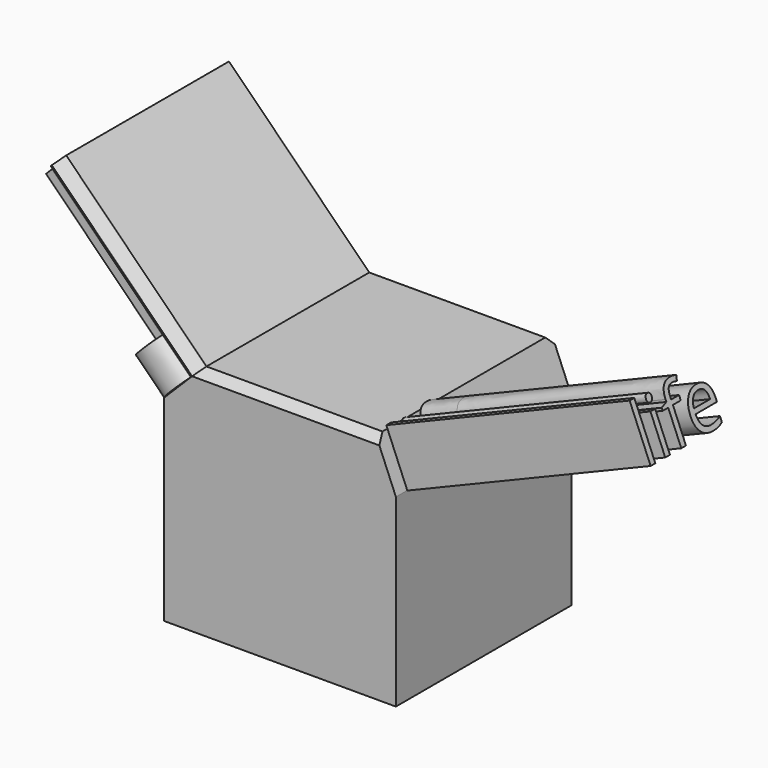
from build123d import *

# Parameters (mm, degrees)
F0_W         = 147.5178673863
F0_H         = 148.0135470629
F1_DEPTH     = 139.7
F2_SIZE      = 22.86
F3_SIZE      = 5.08
F4_TEXT_SIZE = 44.9012806053
F5_DEPTH     = 25.4
F6_T1_DEPTH  = 271.4076559597
F7_TEXT_SIZE = 46.0137451665
F8_DEPTH     = 25.4
F9_DEPTH     = 167.64
F10_DEPTH    = 126.238


# Not quite as in the source:
# - a fillet or chamfer that OpenCascade refuses, or shapes differently, is made with other operations: its cross-section is extruded or revolved along the edge and cut away or added
# - Text() gives the source's letters only with a copy of the font that has no kerning and outlines rounded to 1/6400 em; it was checked with that copy


with BuildPart() as f1:
    # F0 (on Front) → F1 (new body)
    with BuildSketch(Plane.XZ):
        with Locations((-1.3054646552, 0.765427947)):
            Rectangle(F0_W, F0_H)
    extrude(amount=F1_DEPTH)

    # F2
    f2_edges = [f1.edges().sort_by_distance(p)[0] for p in [
        (-75.064398, -69.85, 74.772201),
    ]]
    chamfer(f2_edges, length=F2_SIZE)

    # F3
    f3_edges = [f1.edges().sort_by_distance(p)[0] for p in [
        (10.124535, 0, 74.772201),
        (72.453469, -69.85, 74.772201),
        (10.124535, -139.7, 74.772201),
    ]]
    chamfer(f3_edges, length=F3_SIZE)

    # F4 (on face) → F5 (join)
    with BuildSketch(Plane(origin=(-63.4882999134, 0, 63.4882999134), x_dir=(0, -1, 0), z_dir=(-0.7071067812, 0, 0.7071067812))):
        with Locations((5.08, -16.371075406)):
            Text('trump', F4_TEXT_SIZE, font='Open Sans', font_style=FontStyle.BOLD, text_align=(TextAlign.LEFT, TextAlign.BOTTOM))
    extrude(amount=F5_DEPTH)

    # F6: chamfer of 25.4 on 1 edges, made by hand

    # F6_s2 → F6_t1 (cut)
    with BuildSketch(Plane.XZ.offset(-65.8538279798)):
        Polygon((54.4929567959, 87.6527137206), (72.453469038, 44.2922014785), (72.453469038, 69.6922014785), align=None)
    extrude(amount=F6_T1_DEPTH, mode=Mode.SUBTRACT)

    # F7 (on face) → F8 (join)
    with BuildSketch(Plane(origin=(77.5025621672, 0, 32.1026123683), x_dir=(0, 1, 0), z_dir=(0.9238795325, 0, 0.3826834324))):
        with Locations((-134.62, 13.0553339226)):
            Text('life', F7_TEXT_SIZE, font='Open Sans', text_align=(TextAlign.LEFT, TextAlign.BOTTOM))
    extrude(amount=F8_DEPTH)

    # F7 (on face) → F9 (join)
    with BuildSketch(Plane(origin=(77.5025621672, 0, 32.1026123683), x_dir=(0, 1, 0), z_dir=(0.9238795325, 0, 0.3826834324))):
        with Locations((-134.62, 13.0553339226)):
            Text('life', F7_TEXT_SIZE, font='Open Sans', text_align=(TextAlign.LEFT, TextAlign.BOTTOM))
    extrude(amount=F9_DEPTH)

    # F10 (add): a face of the model
    f10_faces = [f1.faces().sort_by_distance(p)[0] for p in [
        (-61.2852687785, -59.7252792181, 65.6913310483),
    ]]
    extrude(f10_faces, amount=F10_DEPTH)


solid = f1.part
